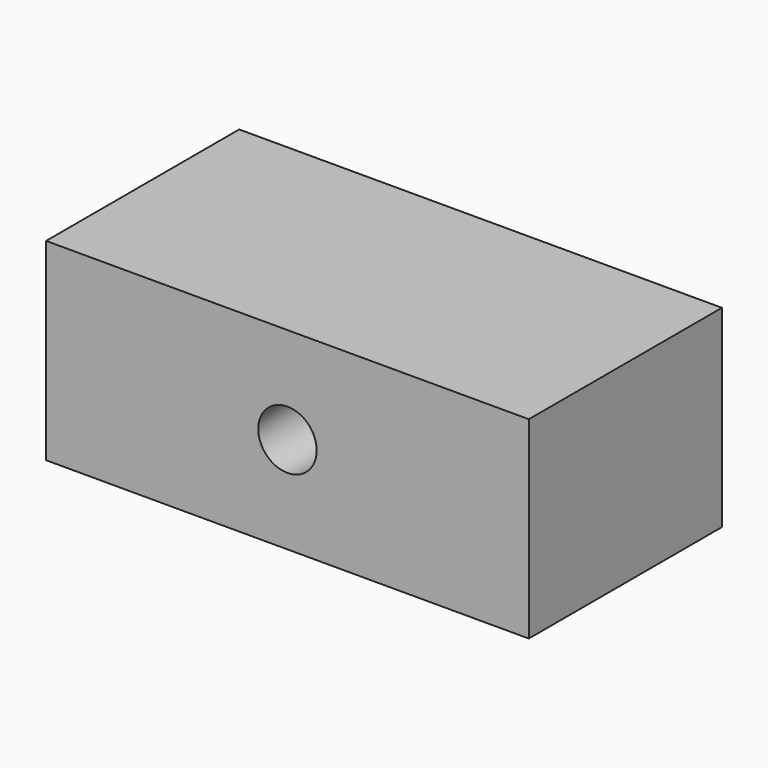
from build123d import *

# Parameters (mm, degrees)
F0_W     = 50
F0_H     = 20
F0_R     = 3.025
F1_DEPTH = 25
F0_R_2   = 1.402
F3_DEPTH = 2


# Not quite as in the source:
# - the program builds the solid bodies; features that only make, move or delete a surface that nothing else refers to are left out


with BuildPart() as f1:
    # F0 (on Front) → F1 (new body)
    with BuildSketch(Plane.XZ):
        Rectangle(F0_W, F0_H)
        Circle(F0_R, mode=Mode.SUBTRACT)
    extrude(amount=F1_DEPTH)


with BuildPart() as f3:
    # F0 (on Front) → F3 (new body)
    with BuildSketch(Plane.XZ):
        Circle(F0_R)
        Circle(F0_R_2, mode=Mode.SUBTRACT)
    extrude(amount=F3_DEPTH)


solid = Compound([f1.part, f3.part])
